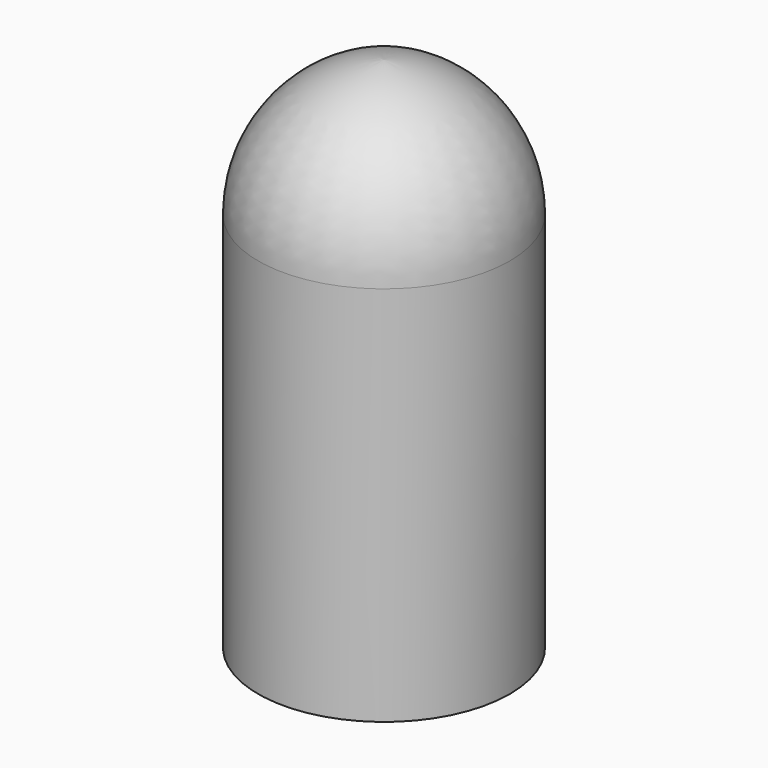
from build123d import *

# Parameters (mm, degrees)
F0_W = 0.381
F0_H = 15.24


# Not quite as in the source:
# - a feature names something its author has since deleted; it is built from what else it names


with BuildPart() as f1:
    # F0 (on Front) → F1 (revolve)
    with BuildSketch(Plane.XZ):
        with BuildLine():
            ThreePointArc((0, 20.3016152323), (3.3098536451, 18.6760483117), (4.6482, 15.24))
            Line((4.6482, 15.24), (5.0292, 15.24))
            ThreePointArc((5.0292, 15.24), (3.5794035834, 18.9452298582), (0, 20.6826152323))
            Line((0, 20.6826152323), (0, 20.3016152323))
        make_face()
        with Locations((4.8387, 7.62)):
            Rectangle(F0_W, F0_H)
    revolve(axis=Axis((0, 0, 8.3369510248), (0, 0, 1)))


solid = f1.part
